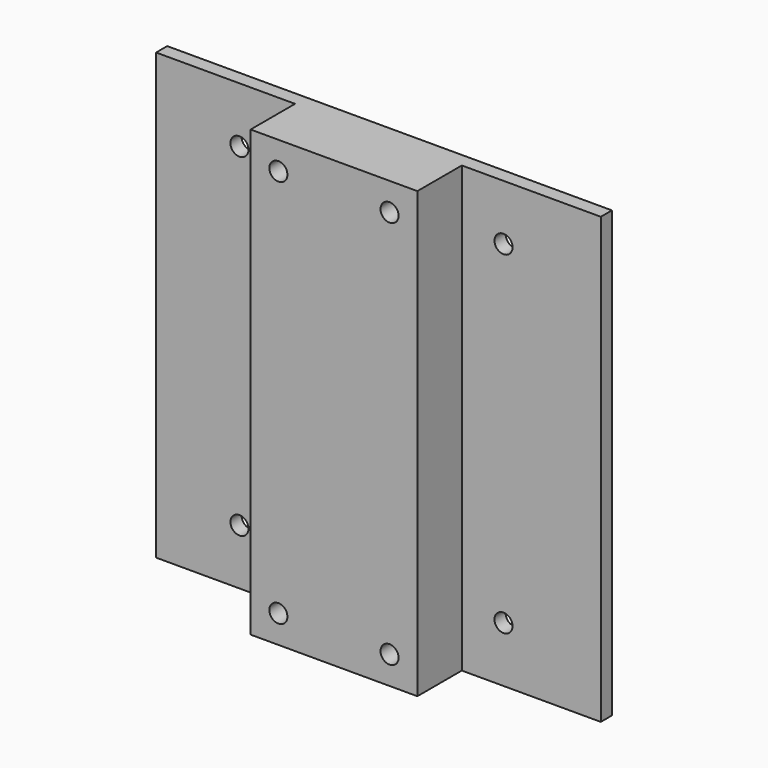
from build123d import *

# Parameters (mm, degrees)
F0_W     = 50
F0_H     = 160
F0_R     = 3.25
F1_DEPTH = 5
F0_W_2   = 60
F2_DEPTH = 25


# Not quite as in the source:
# - a feature names something its author has since deleted; it is built from what else it names


with BuildPart() as f1:
    # F0 (on Front) → F1 (new body)
    with BuildSketch(Plane.XZ):
        with Locations((-52.5, 0)):
            Rectangle(F0_W, F0_H)
        with Locations((-47.5, -60)):
            Circle(F0_R, mode=Mode.SUBTRACT)
        with Locations((-47.5, 60)):
            Circle(F0_R, mode=Mode.SUBTRACT)
    extrude(amount=F1_DEPTH)



with BuildPart() as f1b:
    # F0 (on Front) → F1, piece 2 (new body)
    with BuildSketch(Plane.XZ):
        with Locations((57.5, 0)):
            Rectangle(F0_W, F0_H)
        with Locations((47.5, -60)):
            Circle(F0_R, mode=Mode.SUBTRACT)
        with Locations((47.5, 60)):
            Circle(F0_R, mode=Mode.SUBTRACT)
    extrude(amount=F1_DEPTH)


with BuildPart() as f1_1:
    add(f1.part)

    add(f1b.part)  # F2 merges F1b
    # F0 (on Front) → F2 (join)
    with BuildSketch(Plane.XZ):
        with Locations((2.5, 0)):
            Rectangle(F0_W_2, F0_H)
        with Locations((-17.5, -70)):
            Circle(F0_R, mode=Mode.SUBTRACT)
        with Locations((22.5, -70)):
            Circle(F0_R, mode=Mode.SUBTRACT)
        with Locations((-17.5, 70)):
            Circle(F0_R, mode=Mode.SUBTRACT)
        with Locations((22.5, 70)):
            Circle(F0_R, mode=Mode.SUBTRACT)
    extrude(amount=F2_DEPTH)


solid = f1_1.part
